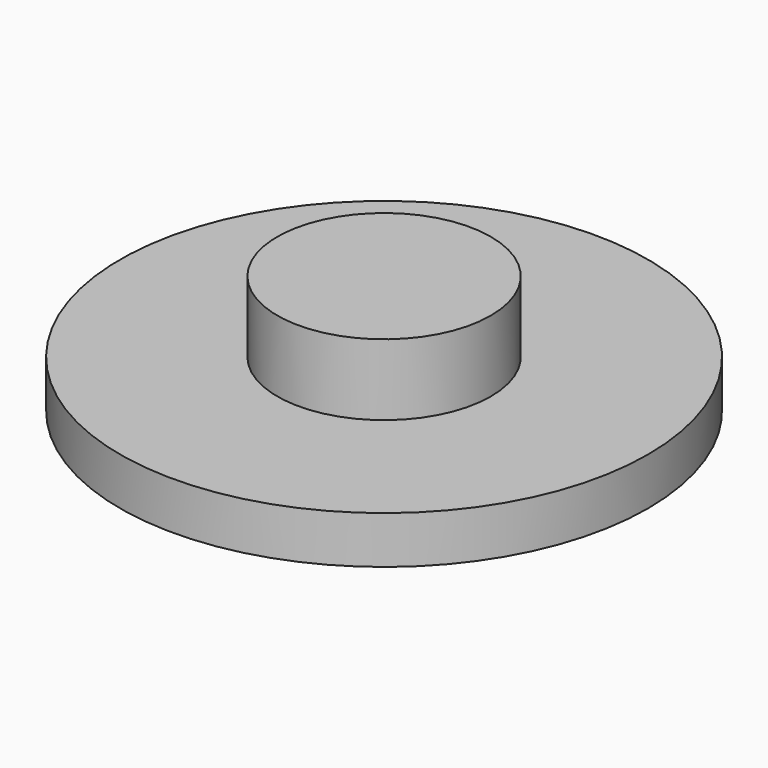
from build123d import *

# Parameters (mm, degrees)
F0_R         = 4.5
F1_DEPTH     = 3
F2_R         = 11.125
F3_DEPTH     = 2
F4_TEXT_SIZE = 21.1666666667
F5_DEPTH     = 0.5


# Not quite as in the source:
# - Text() gives the source's letters only with a copy of the font that has no kerning and outlines rounded to 1/6400 em; it was checked with that copy


with BuildPart() as f1:
    # F0 (on Top) → F1 (new body)
    with BuildSketch(Plane.XY):
        Circle(F0_R)
    extrude(amount=F1_DEPTH)

    # F2 (on Top) → F3 (join)
    with BuildSketch(Plane.XY):
        Circle(F2_R)
    extrude(amount=-F3_DEPTH)

    # F4 (on face) → F5 (cut)
    with BuildSketch(Plane(origin=(0, 0, -2), x_dir=(1, 0, 0), z_dir=(0, 0, -1))):
        with Locations((-8.3393359375, -7.62)):
            Text('N', F4_TEXT_SIZE, font='Open Sans', font_style=FontStyle.BOLD, text_align=(TextAlign.LEFT, TextAlign.BOTTOM))
    extrude(amount=-F5_DEPTH, mode=Mode.SUBTRACT)


solid = f1.part
